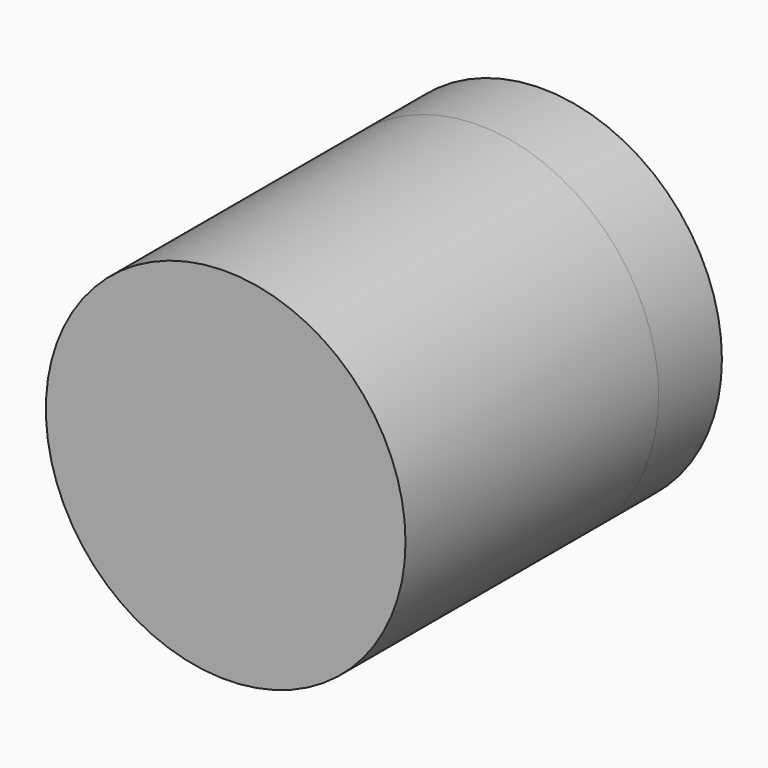
from build123d import *

# Parameters (mm, degrees)
F0_R     = 57.747245906
F1_DEPTH = 25.4
F2_DEPTH = 25.4
F3_DEPTH = 25.4
F4_DEPTH = 25.4
F7_DEPTH = 25.4


# Not quite as in the source:
# - the program builds the solid bodies; features that only make, move or delete a surface that nothing else refers to are left out


with BuildPart() as f1:
    # F0 (on Front) → F1 (new body)
    with BuildSketch(Plane.XZ):
        Circle(F0_R)
    extrude(amount=F1_DEPTH)

    # F2 (add): a face of the model
    f2_faces = [f1.faces().sort_by_distance(p)[0] for p in [
        (0, 0, 0),
    ]]
    extrude(f2_faces, amount=F2_DEPTH)

    # F3 (add): a face of the model
    f3_faces = [f1.faces().sort_by_distance(p)[0] for p in [
        (0, -25.4, 0),
    ]]
    extrude(f3_faces, amount=F3_DEPTH)

    # F4 (add): a face of the model
    f4_faces = [f1.faces().sort_by_distance(p)[0] for p in [
        (0, -50.8, 0),
    ]]
    extrude(f4_faces, amount=F4_DEPTH)

    # F7 (add): a face of the model
    f7_faces = [f1.faces().sort_by_distance(p)[0] for p in [
        (0, 25.4, 0),
    ]]
    extrude(f7_faces, amount=F7_DEPTH)


solid = f1.part
